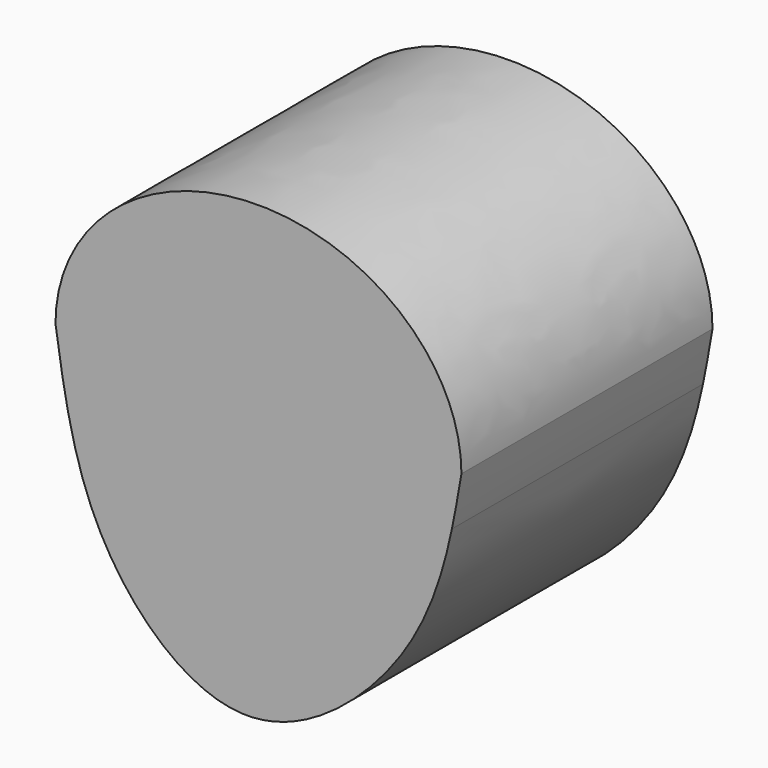
from build123d import *

# Parameters (mm, degrees)
F1_DEPTH = 50.8


with BuildPart() as f1:
    # F0 (on Front) → F1 (new body)
    with BuildSketch(Plane.XZ):
        with BuildLine():
            add(Edge.make_bspline(
                [(26.8634640441, 30.0725474095), (27.4503774573, 32.8547975525), (27.9298393949, 35.6489431931), (28.4093022346, 38.4430885315)],
                knots=[0.9262660757, 0.9262660757, 0.9262660757, 0.9262660757, 1, 1, 1, 1], degree=3))
            add(Edge.make_bspline(
                [(28.4093022346, 38.4430885315), (28.4093022346, 66.056851956), (-4.4455230236, 66.056851956), (-37.3003482819, 66.056851956), (-37.3003482819, 38.4430885315)],
                knots=[0, 0, 0, 1.5707963268, 1.5707963268, 3.1415926536, 3.1415926536, 3.1415926536], degree=2, weights=[1, 0.7071067812, 1, 0.7071067812, 1]))
            add(Edge.make_bspline(
                [(-37.3003482819, 38.4430885315), (-36.939333387, 36.041498013), (-36.5783185118, 33.6399074922), (-36.1667983256, 31.2521979805)],
                knots=[0, 0, 0, 0, 0.0600642843, 0.0600642843, 0.0600642843, 0.0600642843], degree=3))
            add(Edge.make_bspline(
                [(-36.1667983256, 31.2521979805), (-7.0407045556, -59.5095977908), (26.8634640441, 30.0725474095)],
                knots=[3.405039124, 3.405039124, 3.405039124, 5.9752105426, 5.9752105426, 5.9752105426], degree=2, weights=[1, 0.2818393326, 1]))
        make_face()
        with BuildLine():
            add(Edge.make_bspline(
                [(-36.1667983256, 31.2521979805), (-34.8445259273, 23.5801505614), (-30.6813709026, 6.5799650339), (-6.2447021875, -15.5619977157), (20.5872658458, 7.4633058375), (25.4857013307, 23.5412935316), (26.8634640441, 30.0725474095)],
                knots=[0.0600642843, 0.0600642843, 0.0600642843, 0.0600642843, 0.2530593012, 0.4958547101, 0.7531777644, 0.9262660757, 0.9262660757, 0.9262660757, 0.9262660757], degree=3))
            add(Edge.make_bspline(
                [(-36.1667983256, 31.2521979805), (-7.0407045556, -59.5095977908), (26.8634640441, 30.0725474095)],
                knots=[3.405039124, 3.405039124, 3.405039124, 5.9752105426, 5.9752105426, 5.9752105426], degree=2, weights=[1, 0.2818393326, 1]))
        make_face()
    extrude(amount=F1_DEPTH)


solid = f1.part
